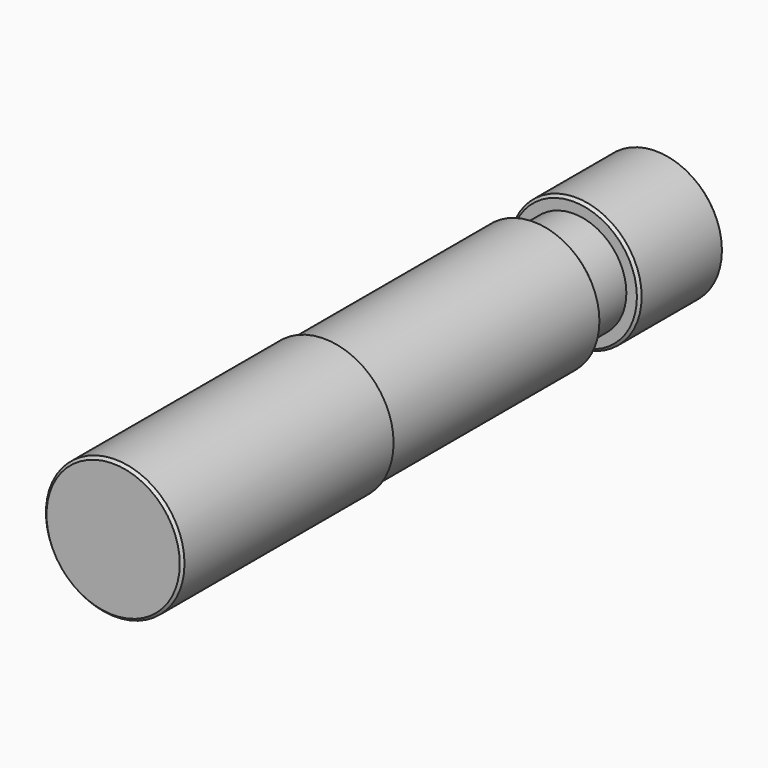
from build123d import *

# Parameters (mm, degrees)
F0_R     = 25
F1_DEPTH = 40
F2_R     = 20
F3_DEPTH = 18
F4_SIZE  = 1
F5_R     = 25
F6_DEPTH = 100
F7_SIZE  = 1
F8_R     = 26.24
F9_DEPTH = 100
F10_SIZE = 1


with BuildPart() as f1:
    # F0 (on Front) → F1 (new body)
    with BuildSketch(Plane.XZ):
        Circle(F0_R)
    extrude(amount=F1_DEPTH)

    # F2 (on face) → F3 (join)
    with BuildSketch(Plane.XZ.offset(40)):
        Circle(F2_R)
    extrude(amount=F3_DEPTH)

    # F4
    f4_edges = [f1.edges().sort_by_distance(p)[0] for p in [
        (-25, -40, 0),
        (-25, 0, 0),
    ]]
    chamfer(f4_edges, length=F4_SIZE)

    # F5 (on face) → F6 (join)
    with BuildSketch(Plane.XZ.offset(58)):
        Circle(F5_R)
    extrude(amount=F6_DEPTH)

    # F7
    f7_edges = [f1.edges().sort_by_distance(p)[0] for p in [
        (-25, -58, 0),
    ]]
    chamfer(f7_edges, length=F7_SIZE)

    # F8 (on face) → F9 (join)
    with BuildSketch(Plane.XZ.offset(158)):
        Circle(F8_R)
    extrude(amount=F9_DEPTH)

    # F10
    f10_edges = [f1.edges().sort_by_distance(p)[0] for p in [
        (-26.24, -258, 0),
    ]]
    chamfer(f10_edges, length=F10_SIZE)


solid = f1.part
